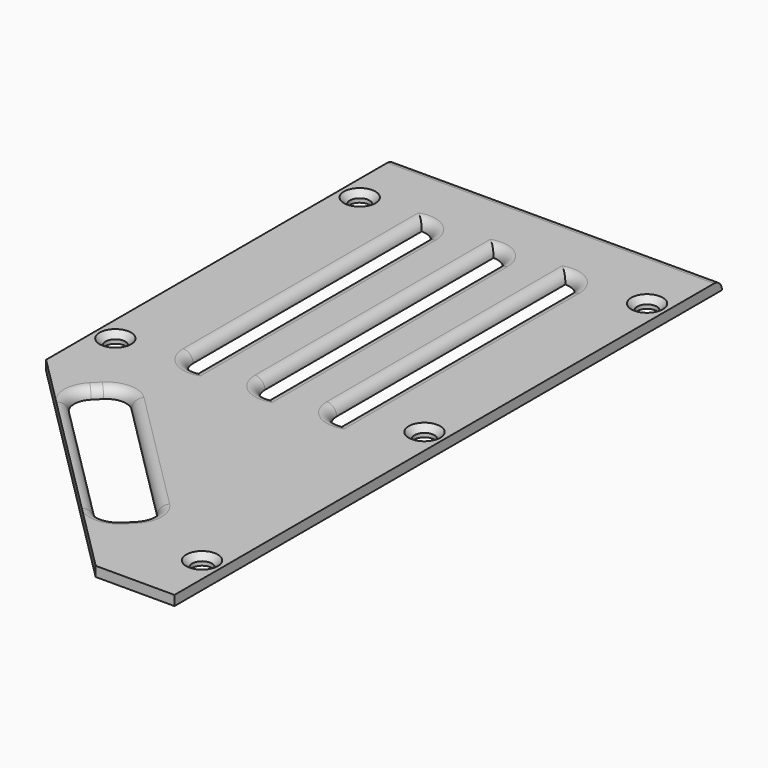
from build123d import *

# Parameters (mm, degrees)
F0_R     = 2.5
F1_DEPTH = 1.25
F2_R     = 2.49999
F3_SIZE  = 1.5


# Not quite as in the source:
# - a fillet or chamfer is up to 0.001 mm smaller than in the source, because OpenCascade refuses the exact size


with BuildPart() as f1:
    # F0 (on Top) → F1 (new body, symmetric)
    with BuildSketch(Plane.XY):
        Polygon((41.4534954924, 86.8201051839), (-41.4535404544, 86.8201051839), (-41.4535404544, -23.9118914119), (21.4531252731, -86.8199001066), (41.4534954924, -86.8199001066), align=None)
        with BuildLine():
            ThreePointArc((-25.0127278268, -26.2106563896), (-21.4771550521, -24.7462917212), (-17.9416265813, -26.210763353))
            Line((-17.9416265813, -26.210763353), (14.5847404845, -58.7378248101))
            ThreePointArc((14.5847404845, -58.7378248101), (16.0492105587, -62.2733815916), (14.5847972009, -65.8089618652))
            Line((14.5847972009, -65.8089618652), (12.816990028, -67.5766218932))
            ThreePointArc((12.816990028, -67.5766218932), (9.2814327639, -69.0409837172), (5.745914741, -67.5765271526))
            Line((5.745914741, -67.5765271526), (-26.7805685052, -35.0493495125))
            ThreePointArc((-26.7805685052, -35.0493495125), (-28.2451162288, -31.5138612573), (-26.7805848271, -27.9783662409))
            Line((-26.7805848271, -27.9783662409), (-25.0127278268, -26.2106563896))
        make_face(mode=Mode.SUBTRACT)
        with Locations((-36.4535404544, -8.1798948161)):
            Circle(F0_R, mode=Mode.SUBTRACT)
        with Locations((36.4534954924, -71.8298948161)):
            Circle(F0_R, mode=Mode.SUBTRACT)
        with Locations((36.4534954924, -1.2798948161)):
            Circle(F0_R, mode=Mode.SUBTRACT)
        with BuildLine():
            Line((-20.7271233506, -3.1984749304), (-20.7271233506, 69.3290029653))
            ThreePointArc((-20.7271233506, 69.3290029653), (-17.1909981799, 67.8582257506), (-15.7271233506, 64.3192375729))
            Line((-15.7271233506, 64.3192375729), (-15.7271233506, -8.1786223686))
            ThreePointArc((-15.7271233506, -8.1786223686), (-19.2614484064, -6.7269968768), (-20.7271233506, -3.1984749304))
        make_face(mode=Mode.SUBTRACT)
        with BuildLine():
            Line((-2.5021233506, -3.1984749304), (-2.5021233506, 69.3290029653))
            ThreePointArc((-2.5021233506, 69.3290029653), (1.0340018201, 67.8582257506), (2.4978766494, 64.3192375729))
            Line((2.4978766494, 64.3192375729), (2.4978766494, -8.1786223686))
            ThreePointArc((2.4978766494, -8.1786223686), (-1.0364484064, -6.7269968768), (-2.5021233506, -3.1984749304))
        make_face(mode=Mode.SUBTRACT)
        with Locations((-36.4535404544, 69.3201051839)):
            Circle(F0_R, mode=Mode.SUBTRACT)
        with BuildLine():
            Line((15.7228766494, -3.1984749304), (15.7228766494, 69.3290029653))
            ThreePointArc((15.7228766494, 69.3290029653), (19.2590018201, 67.8582257506), (20.7228766494, 64.3192375729))
            Line((20.7228766494, 64.3192375729), (20.7228766494, -8.1786223686))
            ThreePointArc((20.7228766494, -8.1786223686), (17.1885515936, -6.7269968768), (15.7228766494, -3.1984749304))
        make_face(mode=Mode.SUBTRACT)
        with Locations((36.4534954924, 69.3201051839)):
            Circle(F0_R, mode=Mode.SUBTRACT)
    extrude(amount=F1_DEPTH, both=True)

    # F2 (radius 2.5 in the source; OpenCascade refuses exactly that, so slightly less here)
    f2_edges = [f1.edges().sort_by_distance(p)[0] for p in [
        (-10.517327, -51.312938, 1.25),
        (-20.727123, 33.065264, 1.25),
        (-2.502123, 33.065264, 1.25),
        (15.722877, 33.065264, 1.25),
        (-17.190998, 67.858226, 1.25),
        (1.034002, 67.858226, 1.25),
        (19.259002, 67.858226, 1.25),
        (-2.2e-05, 86.820105, 1.25),
    ]]
    fillet(f2_edges, radius=F2_R)

    # F3
    f3_edges = [f1.edges().sort_by_distance(p)[0] for p in [
        (-38.95354, -8.179895, 1.25),
        (-38.95354, 69.320105, 1.25),
        (33.953495, 69.320105, 1.25),
        (33.953495, -1.279895, 1.25),
        (33.953495, -71.829895, 1.25),
    ]]
    chamfer(f3_edges, length=F3_SIZE)


solid = f1.part
